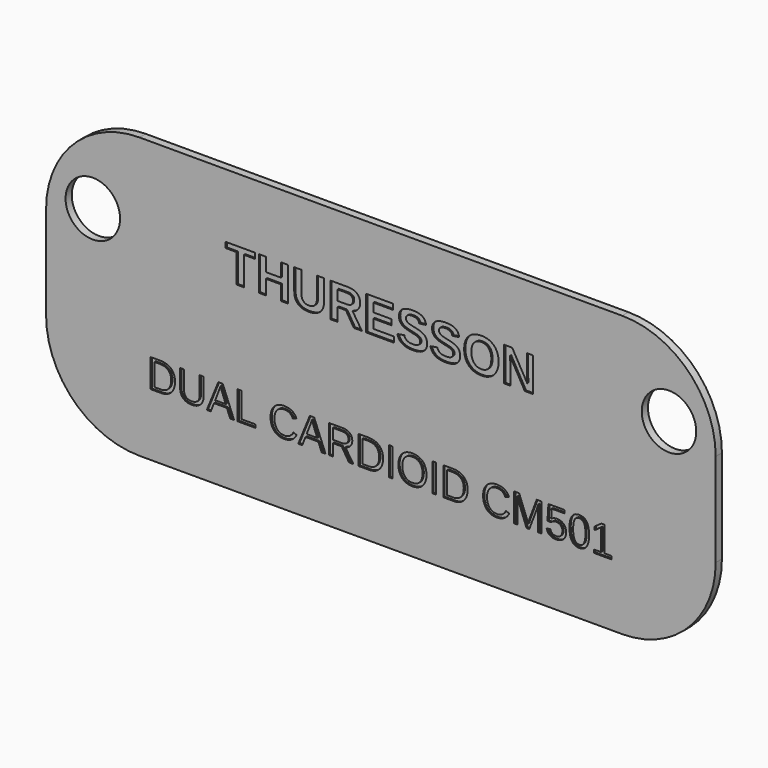
from build123d import *

# Parameters (mm, degrees)
F0_R           = 1.75
F1_DEPTH       = 0.5
F2_TEXT_SIZE   = 3.1844756811
F2_TEXT_SIZE_2 = 2.6416807694
F3_DEPTH       = 0.1


# Not quite as in the source:
# - a feature names something its author has since deleted; it is built from what else it names
# - Text() gives the source's letters only with a copy of the font that has no kerning and outlines rounded to 1/6400 em; it was checked with that copy


with BuildPart() as f1:
    # F0 (on Front) → F1 (new body)
    with BuildSketch(Plane.XZ):
        with BuildLine():
            Line((15.5, 9), (-15.5, 9))
            ThreePointArc((-15.5, 9), (-19.7426406871, 7.2426406871), (-21.5, 3))
            Line((-21.5, 3), (-21.5, -3))
            ThreePointArc((-21.5, -3), (-19.7426406871, -7.2426406871), (-15.5, -9))
            Line((-15.5, -9), (15.5, -9))
            ThreePointArc((15.5, -9), (19.7426406871, -7.2426406871), (21.5, -3))
            Line((21.5, -3), (21.5, 3))
            ThreePointArc((21.5, 3), (19.7426406871, 7.2426406871), (15.5, 9))
        make_face()
        with Locations((-18.5, 4)):
            Circle(F0_R, mode=Mode.SUBTRACT)
        with Locations((18.5, 4)):
            Circle(F0_R, mode=Mode.SUBTRACT)
    extrude(amount=F1_DEPTH)

    # F2 (on face) → F3 (cut)
    with BuildSketch(Plane.XZ.offset(0.5)):
        with Locations((-10, 2.7071775096)):
            Text('THURESSON', F2_TEXT_SIZE, font='Arimo', font_style=FontStyle.BOLD, text_align=(TextAlign.LEFT, TextAlign.BOTTOM))
        with Locations((-15, -5)):
            Text('DUAL CARDIOID CM501', F2_TEXT_SIZE_2, font='Arimo', text_align=(TextAlign.LEFT, TextAlign.BOTTOM))
    extrude(amount=-F3_DEPTH, mode=Mode.SUBTRACT)


solid = f1.part
